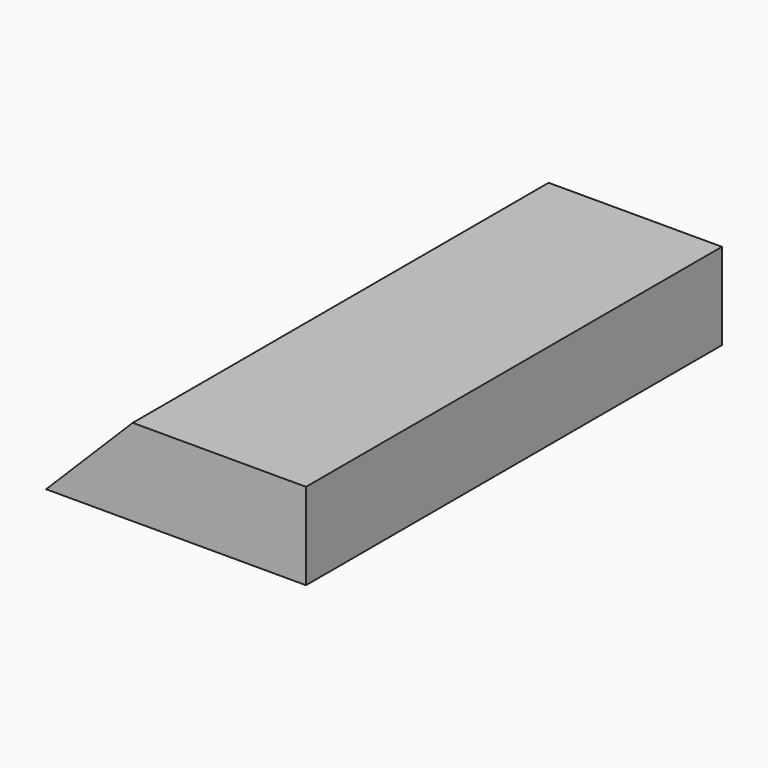
from build123d import *

# Parameters (mm, degrees)
F0_W     = 38.1
F0_H     = 76.2
F1_DEPTH = 12.7
F2_SIZE2 = 12.69999
F2_SIZE  = 12.69999


# Not quite as in the source:
# - a fillet or chamfer is up to 0.001 mm smaller than in the source, because OpenCascade refuses the exact size


with BuildPart() as f1:
    # F0 (on Top) → F1 (new body)
    with BuildSketch(Plane.XY):
        with Locations((4.4191572815, 4.9848316369)):
            Rectangle(F0_W, F0_H)
    extrude(amount=F1_DEPTH)

    # F2 (size 12.7 and 12.7 in the source; OpenCascade refuses exactly that, so slightly less here)
    f2_edges = [f1.edges().sort_by_distance(p)[0] for p in [
        (-14.630843, 4.984832, 12.7),
    ]]
    chamfer(f2_edges, length=F2_SIZE, length2=F2_SIZE2)


solid = f1.part
